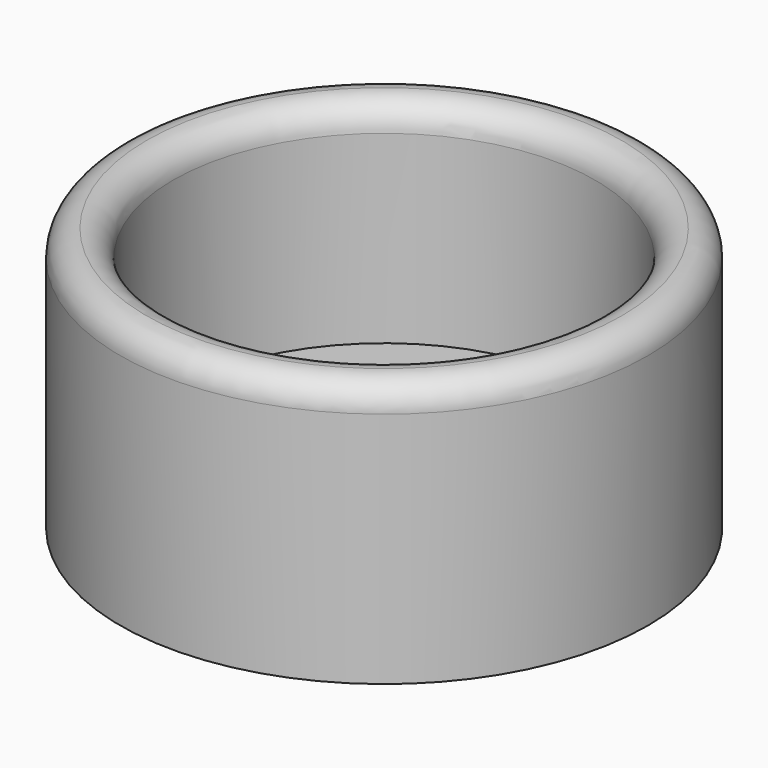
from build123d import *

# Parameters (mm, degrees)
F0_R     = 25
F0_R_2   = 20
F1_DEPTH = 20
F2_R     = 25
F3_DEPTH = 5
F4_R     = 2.5
F5_R     = 2.49999


# Not quite as in the source:
# - a fillet or chamfer is up to 0.001 mm smaller than in the source, because OpenCascade refuses the exact size


with BuildPart() as f1:
    # F0 (on Top) → F1 (new body)
    with BuildSketch(Plane.XY):
        Circle(F0_R)
        Circle(F0_R_2, mode=Mode.SUBTRACT)
    extrude(amount=F1_DEPTH)

    # F2 (on face) → F3 (join)
    with BuildSketch(Plane(origin=(0, 0, 0), x_dir=(1, 0, 0), z_dir=(0, 0, -1))):
        Circle(F2_R)
    extrude(amount=F3_DEPTH)

    # F4
    f4_edges = [f1.edges().sort_by_distance(p)[0] for p in [
        (-25, 0, 20),
    ]]
    fillet(f4_edges, radius=F4_R)

    # F5 (radius 2.5 in the source; OpenCascade refuses exactly that, so slightly less here)
    f5_edges = [f1.edges().sort_by_distance(p)[0] for p in [
        (-20, 0, 20),
    ]]
    fillet(f5_edges, radius=F5_R)


solid = f1.part
